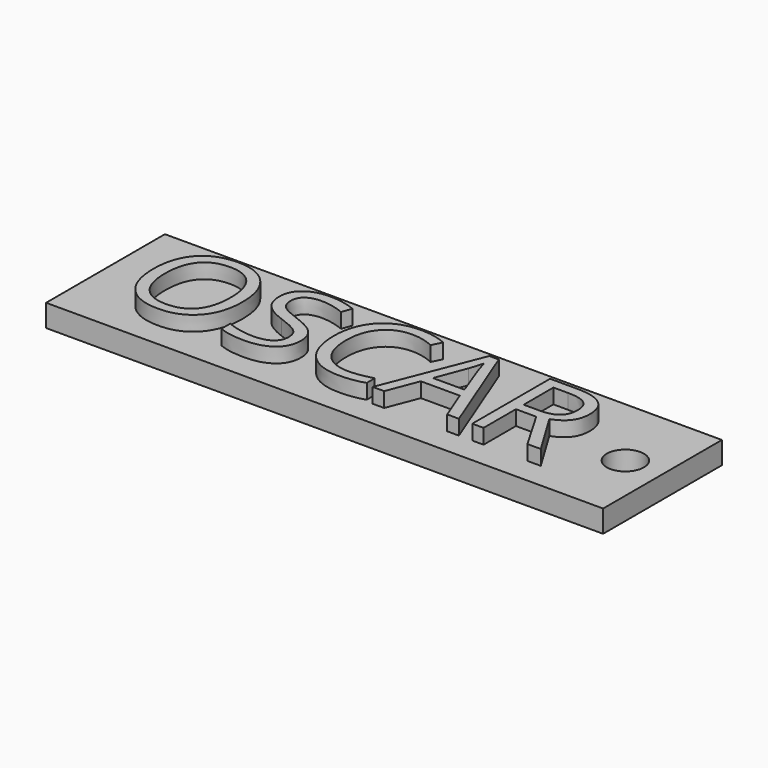
from build123d import *

# Parameters (mm, degrees)
F0_W         = 75
F0_H         = 20
F0_R         = 2.5
F1_DEPTH     = 3
F2_TEXT_SIZE = 18.3423916395
F3_DEPTH     = 2


# Not quite as in the source:
# - Text() gives the source's letters only with a copy of the font that has no kerning and outlines rounded to 1/6400 em; it was checked with that copy


with BuildPart() as f1:
    # F0 (on Top) → F1 (new body)
    with BuildSketch(Plane.XY):
        with Locations((37.5, -10)):
            Rectangle(F0_W, F0_H)
        with Locations((70, -10)):
            Circle(F0_R, mode=Mode.SUBTRACT)
    extrude(amount=F1_DEPTH)

    # F2 (on face) → F3 (join)
    with BuildSketch(Plane.XY.offset(3)):
        with Locations((5.2581620403, -16.5081515443)):
            Text('OSCAR', F2_TEXT_SIZE, font='Open Sans', text_align=(TextAlign.LEFT, TextAlign.BOTTOM))
    extrude(amount=F3_DEPTH)


solid = f1.part
